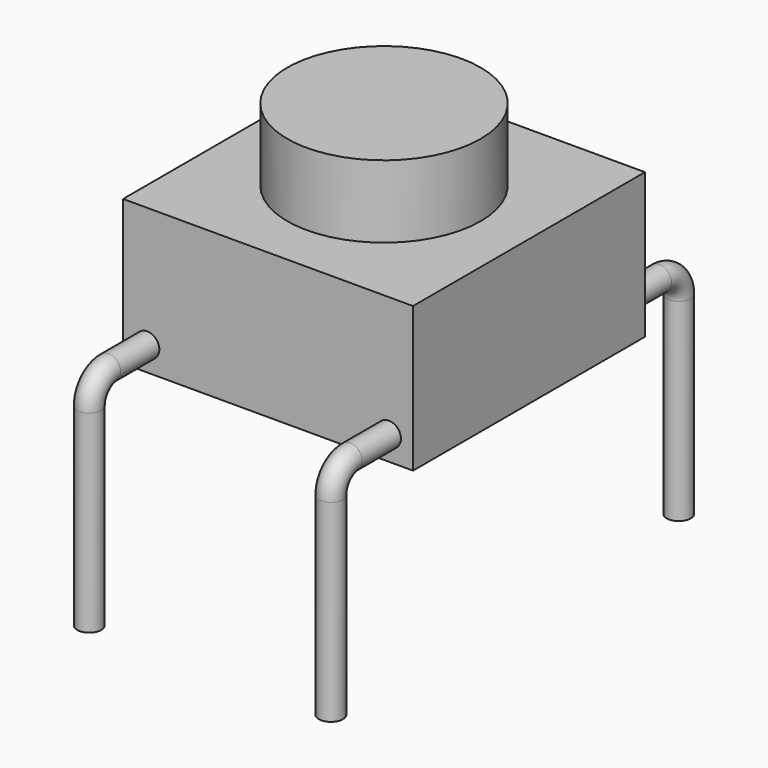
from build123d import *

# Parameters (mm, degrees)
F0_W     = 6
F0_H     = 6
F1_DEPTH = 3
F2_R     = 2
F3_DEPTH = 1.5
F4_R     = 0.25


# Not quite as in the source:
# - a pattern or mirror of a feature is missing from the dataset's text; its kind, count and spacing are read off the source's solid


with BuildPart() as f1:
    # F0 (on Top) → F1 (new body)
    with BuildSketch(Plane.XY):
        Rectangle(F0_W, F0_H)
    extrude(amount=F1_DEPTH)

    # F2 (on face) → F3 (join)
    with BuildSketch(Plane.XY.offset(3)):
        Circle(F2_R)
    extrude(amount=F3_DEPTH)

    # F6: sweep along a path in F5
    with BuildLine(Plane(origin=(-3, 0, 0), x_dir=(0, -1, 0), z_dir=(-1, 0, 0))) as f6_path:
        Line((3, 0.7), (4, 0.7))
        ThreePointArc((4, 0.7), (4.4949747468, 0.4949747468), (4.7, 0))
        Line((4.7, 0), (4.7, -4))
    # F4 (on face) → F6 (sweep)
    with BuildSketch(Plane.XZ.offset(3)):
        with Locations((-2.5, 0.5)):
            Circle(F4_R)
        with Locations((2.5, 0.5)):
            Circle(F4_R)
    f6 = sweep(path=f6_path.line)

    # F6_copies: F6 across plane
    add(f6.mirror(Plane.ZX))


solid = f1.part
